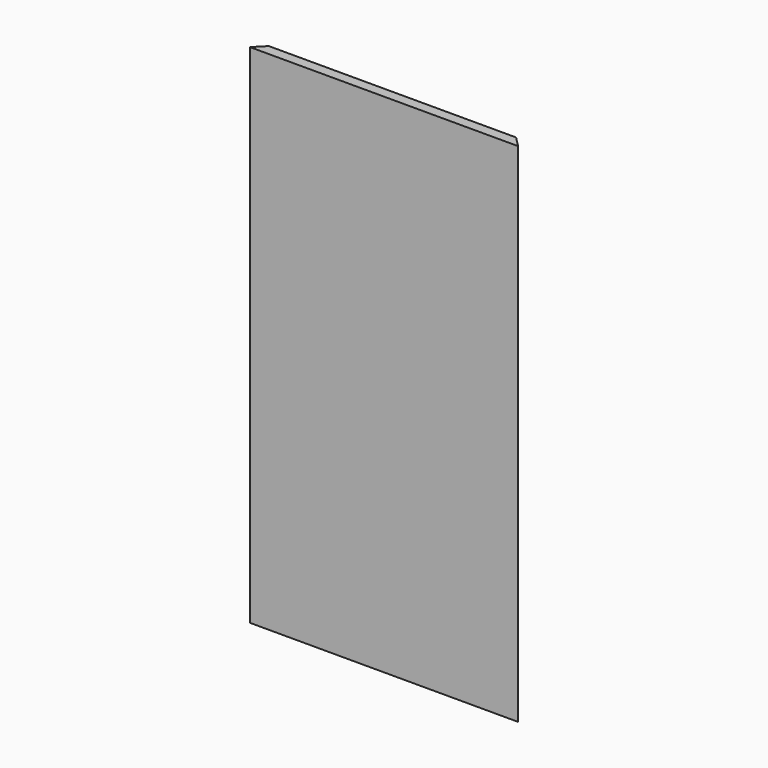
from build123d import *

# Parameters (mm, degrees)
F0_W     = 636.3
F0_H     = 1202
F1_DEPTH = 25
F2_SIZE  = 24.99999


# Not quite as in the source:
# - a fillet or chamfer is up to 0.001 mm smaller than in the source, because OpenCascade refuses the exact size


with BuildPart() as f1:
    # F0 (on Front) → F1 (new body)
    with BuildSketch(Plane.XZ):
        with Locations((318.15, 601)):
            Rectangle(F0_W, F0_H)
    extrude(amount=F1_DEPTH)

    # F2 (size 25 in the source; OpenCascade refuses exactly that, so slightly less here)
    f2_edges = [f1.edges().sort_by_distance(p)[0] for p in [
        (636.3, 0, 601),
        (0, 0, 601),
    ]]
    chamfer(f2_edges, length=F2_SIZE)


solid = f1.part
